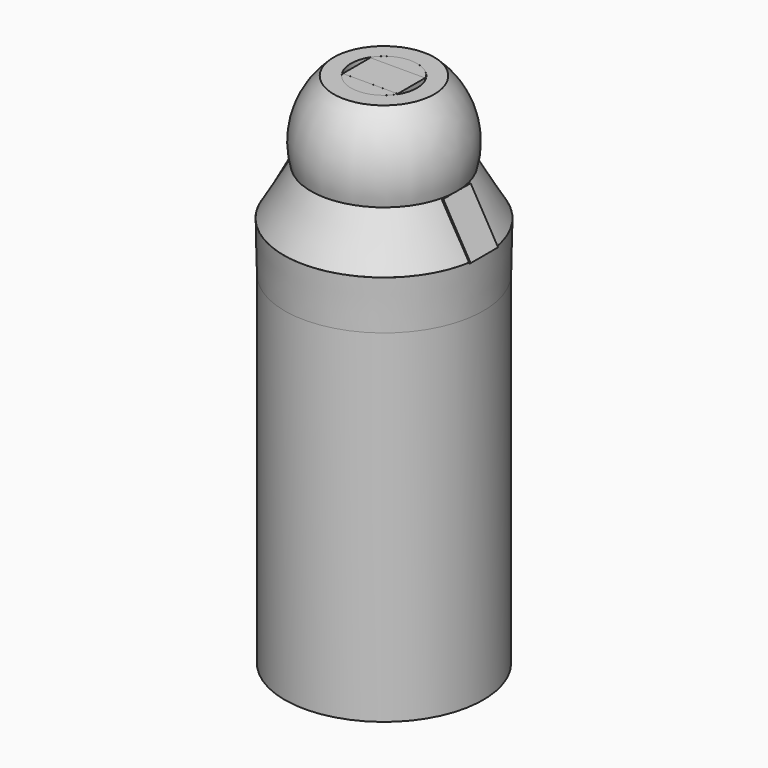
from build123d import *

# Parameters (mm, degrees)
F1_DEPTH = 5
F0_W     = 8
F0_H     = 22
F0_W_2   = 6.7338001877
F0_H_2   = 100
F5_DEPTH = 16
F7_DEPTH = 16


# Not quite as in the source:
# - after a boolean that leaves OpenCascade's solid faulty, fix() repairs it


with BuildPart() as f1:
    # F0 (on Front) → F1 (new body, symmetric)
    with BuildSketch(Plane.XZ):
        Polygon((2.2602713382, 17.2838520708), (10.2602713382, 3.4274456103), (29.3128302215, 14.4274456103), (21.3128302215, 28.2838520708), (9.6675436944, 21.5604427596), align=None)
    extrude(amount=F1_DEPTH, both=True)


with BuildPart() as f1b:
    # F0 (on Front) → F1, piece 2 (new body, symmetric)
    with BuildSketch(Plane.XZ):
        Polygon((-29.3128302215, 14.4274456103), (-10.2602713382, 3.4274456103), (-2.2602713382, 17.2838520708), (-8, 20.5976859588), (-21.3128302215, 28.2838520708), align=None)
    extrude(amount=F1_DEPTH, both=True)


with BuildPart() as f1c:
    # F0 (on Front) → F1, piece 3 (new body, symmetric)
    with BuildSketch(Plane.XZ):
        with Locations((4, 40.0443450212)):
            Rectangle(F0_W, F0_H)
        with Locations((-4, 40.0443450212)):
            Rectangle(F0_W, F0_H)
    extrude(amount=F1_DEPTH, both=True)


with BuildPart() as f2:
    # F0 (on Front) → F2 (revolve)
    with BuildSketch(Plane.XZ):
        with Locations((-25.6330999061, -50)):
            Rectangle(F0_W_2, F0_H_2)
    revolve(axis=Axis((0, 0, -50), (0, 0, -1)))


with BuildPart() as f3:
    # F0 (on Front) → F3 (revolve)
    with BuildSketch(Plane.XZ):
        with BuildLine():
            Line((9.6675436944, 21.5604427596), (21.3128302215, 28.2838520708))
            ThreePointArc((21.3128302215, 28.2838520708), (21.1730407744, 40.5964594654), (14.6567896008, 51.0443450212))
            Line((14.6567896008, 51.0443450212), (9.6675436944, 51.0443450212))
            Line((9.6675436944, 51.0443450212), (9.6675436944, 21.5604427596))
        make_face()
    revolve(axis=Axis((0, 0, 14.5221725106), (0, 0, -1)))


with BuildPart() as f5:
    # F4 (on Top) → F5 (new body)
    with BuildSketch(Plane.XY):
        with BuildLine():
            ThreePointArc((-8.2867536694, -4.938212689), (-0.0331071205, -9.7356702002), (8.2205394283, -4.938212689))
            Line((8.2205394283, -4.938212689), (-8.2867536694, -4.938212689))
        make_face()
    extrude(amount=F5_DEPTH)


with BuildPart() as f5_1:
    # F6: moved
    add(f5.part.moved(Location((0, 0, 35.04))))


with BuildPart() as f7:
    # F4 (on Top) → F7 (new body)
    with BuildSketch(Plane.XY):
        with BuildLine():
            Line((-8.2867536694, 4.938212689), (8.2205394283, 4.938212689))
            ThreePointArc((8.2205394283, 4.938212689), (-0.0331071205, 9.7356702002), (-8.2867536694, 4.938212689))
        make_face()
    extrude(amount=F7_DEPTH)


with BuildPart() as f7_1:
    # F8: moved
    add(f7.part.moved(Location((0, 0, 35.04))))


with BuildPart() as f9:
    # F0 (on Front) → F9 (revolve)
    with BuildSketch(Plane.XZ):
        Polygon((-10.2602713382, 0), (-10.2602713382, 3.4274456103), (-29.3128302215, 14.4274456103), (-29, 0), (-22.2661998123, 0), align=None)
    revolve(axis=Axis((0, 0, 25.5221725106), (0, 0, 1)))


with BuildPart() as f10:
    # F0 (on Front) → F10 (revolve)
    with BuildSketch(Plane.XZ):
        Polygon((-10.2602713382, 0), (-10.2602713382, 3.4274456103), (-29.3128302215, 14.4274456103), (-29, 0), (-22.2661998123, 0), align=None)
    revolve(axis=Axis((0, 0, -50), (0, 0, -1)))


with BuildPart() as f11:
    # F0 (on Front) → F11 (revolve)
    with BuildSketch(Plane.XZ):
        Polygon((2.2602713382, 17.2838520708), (10.2602713382, 3.4274456103), (29.3128302215, 14.4274456103), (21.3128302215, 28.2838520708), (9.6675436944, 21.5604427596), align=None)
    revolve(axis=Axis((0, 0, 25.5221725106), (0, 0, 1)))

    add(f11.part.fix(), mode=Mode.REPLACE)


solid = Compound([f1.part, f1b.part, f1c.part, f2.part, f3.part, f5_1.part, f7_1.part, f9.part, f10.part, f11.part])
